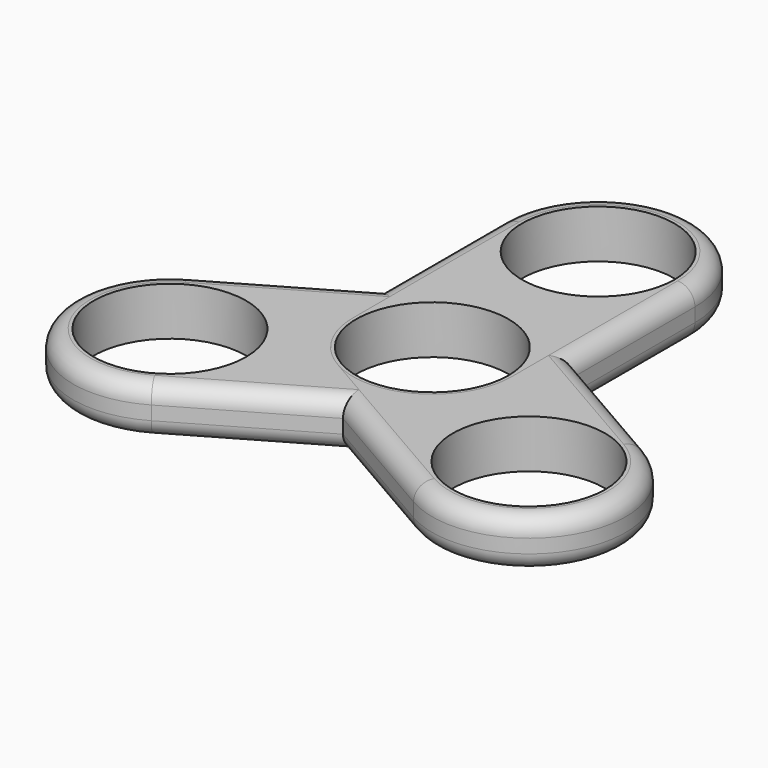
from build123d import *

# Parameters (mm, degrees)
F1_DEPTH        = 7
F1_COPIES_COUNT = 3
F3_R            = 2.5
F3_2_R          = 2.5
F3_3_R          = 2.5


# Not quite as in the source:
# - a feature of the source that left no trace in its solid (it failed there, or was rolled back) is left out
# - a pattern or mirror of a feature is missing from the dataset's text; its kind, count and spacing are read off the source's solid


with BuildPart() as f1:
    # F0 (on Top) → F1 (new body)
    with BuildSketch(Plane.XY):
        with BuildLine():
            Line((11.025, 15), (14, 15))
            ThreePointArc((14, 15), (0, 29), (-14, 15))
            Line((-14, 15), (-11.025, 15))
            ThreePointArc((-11.025, 15), (0, 26.025), (11.025, 15))
        make_face()
        with BuildLine():
            ThreePointArc((-14, 15), (0, 1), (14, 15))
            Line((14, 15), (11.025, 15))
            ThreePointArc((11.025, 15), (0, 3.975), (-11.025, 15))
            Line((-11.025, 15), (-14, 15))
        make_face()
        with BuildLine():
            ThreePointArc((-14, -15), (0, -1), (14, -15))
            Line((14, -15), (14, 15))
            ThreePointArc((14, 15), (0, 1), (-14, 15))
            Line((-14, 15), (-14, -15))
        make_face()
        with BuildLine():
            Line((11.025, -15), (14, -15))
            ThreePointArc((14, -15), (0, -1), (-14, -15))
            Line((-14, -15), (-11.025, -15))
            ThreePointArc((-11.025, -15), (0, -3.975), (11.025, -15))
        make_face()
        with BuildLine():
            ThreePointArc((-14, -15), (0, -29), (14, -15))
            Line((14, -15), (11.025, -15))
            ThreePointArc((11.025, -15), (0, -26.025), (-11.025, -15))
            Line((-11.025, -15), (-14, -15))
        make_face()
    extrude(amount=F1_DEPTH)


with BuildPart() as f1_copies_1:
    # F1_copies: instance of F1
    add(f1.part.rotate(Axis((0, -15, 0), (0, 0, 1)), 1 * 360 / F1_COPIES_COUNT))

    # F3#2
    f3_2_edges = [f1_copies_1.edges().sort_by_distance(p)[0] for p in [
        (-38.105118, -37, 0),
        (-38.105118, -37, 7),
        (-5.990381, -34.624356, 0),
        (-5.990381, -34.624356, 7),
        (-19.990381, -10.375644, 0),
        (-19.990381, -10.375644, 7),
    ]]
    fillet(f3_2_edges, radius=F3_2_R)


with BuildPart() as f1_copies_2:
    # F1_copies: instance of F1
    add(f1.part.rotate(Axis((0, -15, 0), (0, 0, 1)), 2 * 360 / F1_COPIES_COUNT))

    # F3#3
    f3_3_edges = [f1_copies_2.edges().sort_by_distance(p)[0] for p in [
        (38.105118, -37, 0),
        (38.105118, -37, 7),
        (19.990381, -10.375644, 0),
        (19.990381, -10.375644, 7),
        (5.990381, -34.624356, 0),
        (5.990381, -34.624356, 7),
    ]]
    fillet(f3_3_edges, radius=F3_3_R)


with BuildPart() as f1_1:
    add(f1.part)

    # F3
    f3_edges = [f1_1.edges().sort_by_distance(p)[0] for p in [
        (-14, 0, 7),
        (0, 29, 7),
        (14, 0, 7),
        (-14, 0, 0),
        (0, 29, 0),
        (14, 0, 0),
    ]]
    fillet(f3_edges, radius=F3_R)


solid = Compound([f1_copies_1.part, f1_copies_2.part, f1_1.part])
